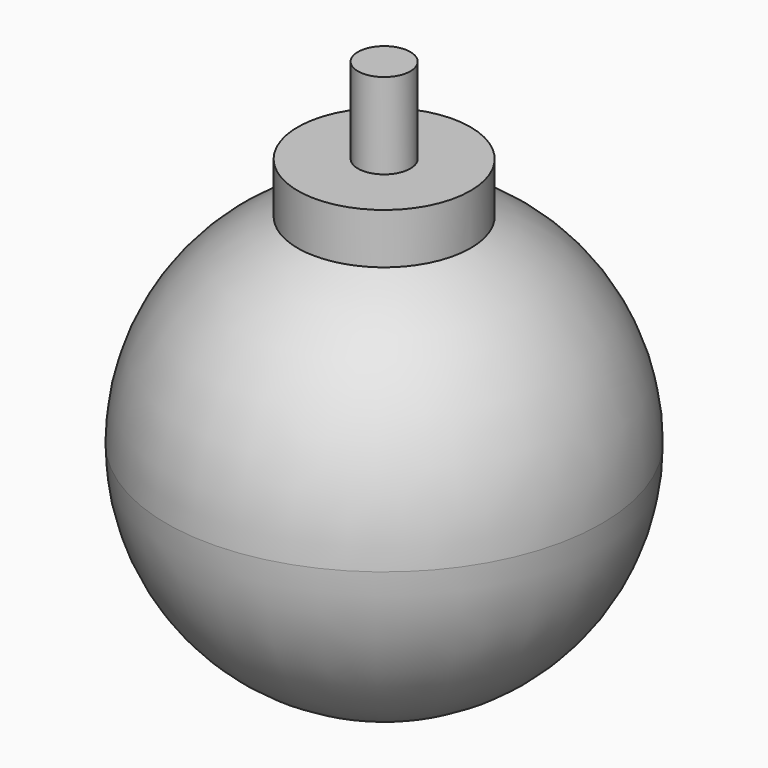
from build123d import *

# Parameters (mm, degrees)
F0_R     = 25.4
F1_DEPTH = 50.8
F2_R     = 25.39999
F4_R     = 10.0773123243
F5_DEPTH = 6.35
F7_R     = 3.0594191455
F8_DEPTH = 10


# Not quite as in the source:
# - a fillet or chamfer is up to 0.001 mm smaller than in the source, because OpenCascade refuses the exact size


with BuildPart() as f1:
    # F0 (on Top) → F1 (new body)
    with BuildSketch(Plane.XY):
        Circle(F0_R)
    extrude(amount=F1_DEPTH)

    # F2 (radius 25.4 in the source; OpenCascade refuses exactly that, so slightly less here)
    f2_edges = [f1.edges().sort_by_distance(p)[0] for p in [
        (-25.4, 0, 50.8),
        (-25.4, 0, 0),
    ]]
    fillet(f2_edges, radius=F2_R)

    # F4 (on offset) → F5 (join)
    with BuildSketch(Plane.XY.offset(48.26)):
        Circle(F4_R)
    extrude(amount=F5_DEPTH)

    # F7 (on offset) → F8 (join)
    with BuildSketch(Plane.XY.offset(54.61)):
        Circle(F7_R)
    extrude(amount=F8_DEPTH)


solid = f1.part
